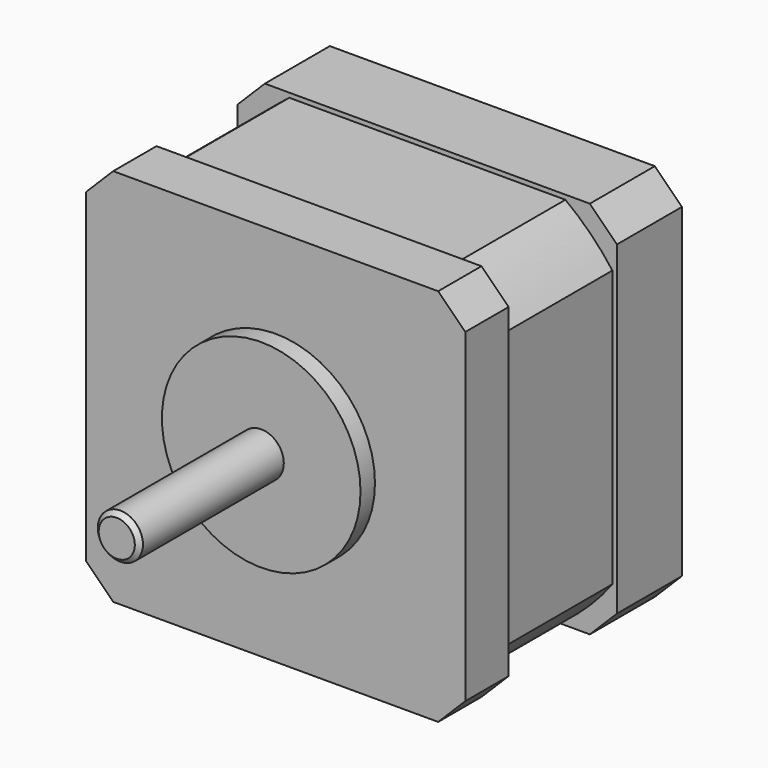
from build123d import *

# Parameters (mm, degrees)
F0_W      = 42
F0_H      = 42
F1_DEPTH  = 9
F2_SIZE   = 3
F3_R      = 15
F4_DEPTH  = 15
F6_DEPTH  = 6
F7_R      = 11
F8_DEPTH  = 2
F9_R      = 2.5
F10_DEPTH = 20
F11_SIZE  = 0.5


with BuildPart() as f1:
    # F0 (on Front) → F1 (new body)
    with BuildSketch(Plane.XZ):
        Rectangle(F0_W, F0_H)
    extrude(amount=F1_DEPTH)

    # F2
    f2_edges = [f1.edges().sort_by_distance(p)[0] for p in [
        (-21, -4.5, 21),
        (21, -4.5, 21),
        (21, -4.5, -21),
        (-21, -4.5, -21),
    ]]
    chamfer(f2_edges, length=F2_SIZE)


with BuildPart() as f4:
    # F3 (on face) → F4 (new body)
    with BuildSketch(Plane.XZ.offset(9)):
        with BuildLine():
            Line((15.2951411283, 20.5), (-15.2951411283, 20.5))
            ThreePointArc((-15.2951411283, 20.5), (-18.0857864376, 18.0857864376), (-20.5, 15.2951411283))
            Line((-20.5, 15.2951411283), (-20.5, -15.2951411283))
            ThreePointArc((-20.5, -15.2951411283), (-18.0857864376, -18.0857864376), (-15.2951411283, -20.5))
            Line((-15.2951411283, -20.5), (15.2951411283, -20.5))
            ThreePointArc((15.2951411283, -20.5), (18.0857864376, -18.0857864376), (20.5, -15.2951411283))
            Line((20.5, -15.2951411283), (20.5, 15.2951411283))
            ThreePointArc((20.5, 15.2951411283), (18.0857864376, 18.0857864376), (15.2951411283, 20.5))
        make_face()
        Circle(F3_R, mode=Mode.SUBTRACT)
        Circle(F3_R)
    extrude(amount=F4_DEPTH)


with BuildPart() as f6:
    # F5 (on face) → F6 (new body)
    with BuildSketch(Plane.XZ.offset(24)):
        Polygon((-18, 21), (-21, 18), (-21, -18), (-18, -21), (18, -21), (21, -18), (21, 18), (18, 21), align=None)
    extrude(amount=F6_DEPTH)

    # F7 (on face) → F8 (join)
    with BuildSketch(Plane.XZ.offset(30)):
        Circle(F7_R)
    extrude(amount=F8_DEPTH)


with BuildPart() as f10:
    # F9 (on face) → F10 (new body)
    with BuildSketch(Plane.XZ.offset(32)):
        Circle(F9_R)
    extrude(amount=F10_DEPTH)

    # F11
    f11_edges = [f10.edges().sort_by_distance(p)[0] for p in [
        (-2.5, -52, 0),
    ]]
    chamfer(f11_edges, length=F11_SIZE)


solid = Compound([f1.part, f4.part, f6.part, f10.part])
